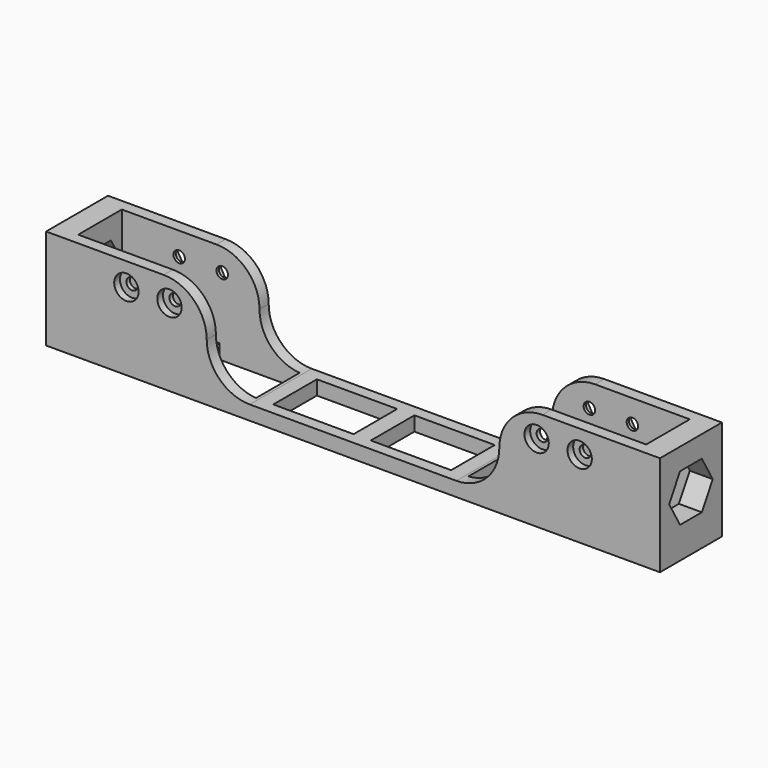
from build123d import *

# Parameters (mm, degrees)
F0_W           = 28
F0_H           = 19
F0_W_2         = 6
F1_DEPTH       = 5
F2_DEPTH       = 30
F3_R           = 14.99999
F6_D           = 4
F6_CBORE_D     = 8.5
F6_CBORE_DEPTH = 2.5
F7_R           = 2
F8_DEPTH       = 3
F10_DEPTH      = 214.001


# Not quite as in the source:
# - a fillet or chamfer is up to 0.001 mm smaller than in the source, because OpenCascade refuses the exact size
# - a feature names something its author has since deleted; it is built from what else it names


with BuildPart() as f1:
    # F0 (on Top) → F1 (new body)
    with BuildSketch(Plane.XY):
        Polygon((-107, 13.5), (-107, -13.5), (-51, -13.5), (-51, -9.5), (-65, -9.5), (-71, -9.5), (-99, -9.5), (-99, 9.5), (-71, 9.5), (-65, 9.5), (-51, 9.5), (-51, 13.5), align=None)
        Polygon((-51, -9.5), (-51, -13.5), (51, -13.5), (51, -9.5), (37, -9.5), (37, 9.5), (51, 9.5), (51, 13.5), (-51, 13.5), (-51, 9.5), (-37, 9.5), (-37, -9.5), align=None)
        with Locations((-17, 0)):
            Rectangle(F0_W, F0_H, mode=Mode.SUBTRACT)
        with Locations((17, 0)):
            Rectangle(F0_W, F0_H, mode=Mode.SUBTRACT)
        Polygon((51, -9.5), (51, -13.5), (107, -13.5), (107, 13.5), (51, 13.5), (51, 9.5), (65, 9.5), (71, 9.5), (99, 9.5), (99, -9.5), (71, -9.5), (65, -9.5), align=None)
        with Locations((-68, 0)):
            Rectangle(F0_W_2, F0_H)
        with Locations((68, 0)):
            Rectangle(F0_W_2, F0_H)
    extrude(amount=-F1_DEPTH)

    # F0 (on Top) → F2 (join)
    with BuildSketch(Plane.XY):
        Polygon((51, -9.5), (51, -13.5), (107, -13.5), (107, 13.5), (51, 13.5), (51, 9.5), (65, 9.5), (71, 9.5), (99, 9.5), (99, -9.5), (71, -9.5), (65, -9.5), align=None)
        Polygon((-107, 13.5), (-107, -13.5), (-51, -13.5), (-51, -9.5), (-65, -9.5), (-71, -9.5), (-99, -9.5), (-99, 9.5), (-71, 9.5), (-65, 9.5), (-51, 9.5), (-51, 13.5), align=None)
    extrude(amount=F2_DEPTH)

    # F3 (radius 15 in the source; OpenCascade refuses exactly that, so slightly less here)
    f3_edges = [f1.edges().sort_by_distance(p)[0] for p in [
        (51, 11.5, 0),
        (51, 11.5, 30),
        (-51, 11.5, 30),
        (-51, 11.5, 0),
        (-51, -11.5, 30),
        (51, -11.5, 30),
    ]]
    fillet(f3_edges, radius=F3_R)

    # F6 (through all)
    with Locations(Plane.XZ.offset(13.5)):
        with Locations((-79, 22), (79, 22), (-64, 22), (64, 22)):
            CounterBoreHole(F6_D / 2, F6_CBORE_D / 2, F6_CBORE_DEPTH)

    # F7 (on face) → F8 (cut)
    with BuildSketch(Plane(origin=(0, 13.5, 0), x_dir=(-1, 0, 0), z_dir=(0, 1, 0))):
        Polygon((-81.1656275844, 18.1837989441), (-76.7778867319, 18.2164109688), (-74.6122591474, 22.0326120247), (-76.8343724156, 25.8162010559), (-81.2221132681, 25.7835890312), (-83.3877408526, 21.9673879753), align=None)
        with Locations((-79, 22)):
            Circle(F7_R, mode=Mode.SUBTRACT)
        Polygon((-59.6121379542, 22), (-61.8060689771, 25.8), (-66.1939310229, 25.8), (-68.3878620458, 22), (-66.1939310229, 18.2), (-61.8060689771, 18.2), align=None)
        with Locations((-64, 22)):
            Circle(F7_R, mode=Mode.SUBTRACT)
        Polygon((61.8060689771, 18.2), (66.1939310229, 18.2), (68.3878620458, 22), (66.1939310229, 25.8), (61.8060689771, 25.8), (59.6121379542, 22), align=None)
        with Locations((64, 22)):
            Circle(F7_R, mode=Mode.SUBTRACT)
        Polygon((76.7778867319, 18.2164109688), (81.1656275844, 18.1837989441), (83.3877408526, 21.9673879753), (81.2221132681, 25.7835890312), (76.8343724156, 25.8162010559), (74.6122591474, 22.0326120247), align=None)
        with Locations((79, 22)):
            Circle(F7_R, mode=Mode.SUBTRACT)
    extrude(amount=-F8_DEPTH, mode=Mode.SUBTRACT)

    # F9 (on face) → F10 (cut, through all)
    with BuildSketch(Plane(origin=(-107, 0, 0), x_dir=(0, -1, 0), z_dir=(-1, 0, 0))):
        Polygon((-4.75, 6), (4.75, 6), (9.5, 14.227241336), (4.75, 22.4544826719), (-4.75, 22.4544826719), (-9.5, 14.227241336), align=None)
    extrude(amount=-F10_DEPTH, mode=Mode.SUBTRACT)


solid = f1.part
